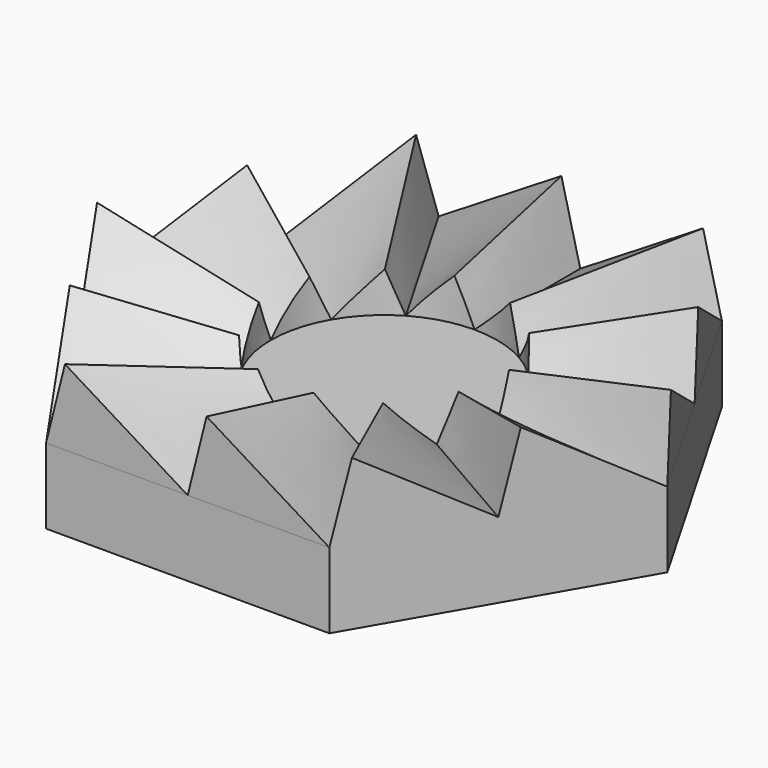
from build123d import *

# Parameters (mm, degrees)
F1_DEPTH        = 2
F6_COPIES_COUNT = 6
F7_COPIES_COUNT = 6
F8_R            = 4
F9_DEPTH        = 1.5
F10_R           = 3
F11_DEPTH       = 2.0010001


# Not quite as in the source:
# - a pattern or mirror of a feature is missing from the dataset's text; its kind, count and spacing are read off the source's solid


with BuildPart() as f1:
    # F0 (on Top) → F1 (new body)
    with BuildSketch(Plane.XY):
        Polygon((3.7527767497, 6.5), (-3.7527767497, 6.5), (-7.5055534995, 0), (-3.7527767497, -6.5), (3.7527767497, -6.5), (7.5055534995, 0), align=None)
    extrude(amount=F1_DEPTH)

    # F5 (on offset) → F6 section 0
    with BuildSketch(Plane(origin=(-2.1650635095, -1.25, 0), x_dir=(0.5, -0.8660254038, 0), z_dir=(-0.8660254038, -0.5, 0))):
        Polygon((-0.943375673, 3), (-1.443375673, 2), (0, 2), align=None)
    # F3 (on face) → F6 section 1
    with BuildSketch(Plane(origin=(-5.6291651246, -3.25, 0), x_dir=(0.5, -0.8660254038, 0), z_dir=(-0.8660254038, -0.5, 0))):
        Polygon((-3.2527767497, 4), (-3.7527767497, 2), (0, 2), align=None)
    f6 = loft()

    # F6_copies: F6 ×6 about axis
    f6_copies_axis = Axis((0, 0, 0), (0, 0, 1))
    for i in range(1, F6_COPIES_COUNT):
        add(f6.rotate(f6_copies_axis, i * 360 / F6_COPIES_COUNT))

    # F5 (on offset) → F7 section 0
    with BuildSketch(Plane(origin=(-2.1650635095, -1.25, 0), x_dir=(0.5, -0.8660254038, 0), z_dir=(-0.8660254038, -0.5, 0))):
        Polygon((0.5, 3), (0, 2), (1.443375673, 2), align=None)
    # F3 (on face) → F7 section 1
    with BuildSketch(Plane(origin=(-5.6291651246, -3.25, 0), x_dir=(0.5, -0.8660254038, 0), z_dir=(-0.8660254038, -0.5, 0))):
        Polygon((0.5, 4), (0, 2), (3.7527767497, 2), align=None)
    f7 = loft()

    # F7_copies: F7 ×6 about axis
    f7_copies_axis = Axis((0, 0, 0), (0, 0, 1))
    for i in range(1, F7_COPIES_COUNT):
        add(f7.rotate(f7_copies_axis, i * 360 / F7_COPIES_COUNT))

    # F8 (on Top) → F9 (cut)
    with BuildSketch(Plane.XY):
        Circle(F8_R)
    extrude(amount=F9_DEPTH, mode=Mode.SUBTRACT)

    # F10 (on face) → F11 (cut, through all)
    with BuildSketch(Plane.XY.offset(2)):
        Circle(F10_R)
    extrude(amount=F11_DEPTH, mode=Mode.SUBTRACT)


solid = f1.part
